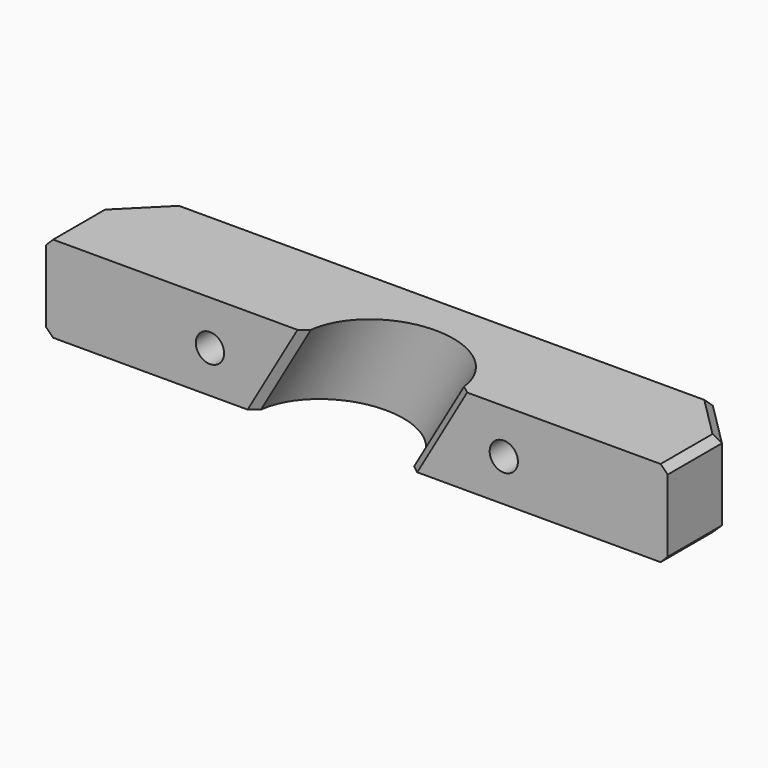
from build123d import *

# Parameters (mm, degrees)
F0_W         = 34.925
F0_H         = 12.7
F1_DEPTH     = 9.7155
F3_R         = 1.5875
F4_DEPTH     = 25.4
F5_SIZE      = 0.79375
F6_T1_DEPTH  = 34.2562991577
F7_SIZE      = 0.79375
F11_R        = 7.493
F12_DEPTH    = 50.8
F13_T1_DEPTH = 15.1455192093
F13_T3_DEPTH = 15.1455192093


# Not quite as in the source:
# - a fillet or chamfer that OpenCascade refuses, or shapes differently, is made with other operations: its cross-section is extruded or revolved along the edge and cut away or added


with BuildPart() as f1:
    # F0 (on Top) → F1 (new body)
    with BuildSketch(Plane.XY):
        with Locations((-17.4625, 6.35)):
            Rectangle(F0_W, F0_H)
        with Locations((17.4625, 6.35)):
            Rectangle(F0_W, F0_H)
    extrude(amount=F1_DEPTH)

    # F3 (on face) → F4 (cut)
    with BuildSketch(Plane(origin=(0, 12.7, 0), x_dir=(-1, 0, 0), z_dir=(0, 1, 0))):
        with Locations((16.51, 4.71678)):
            Circle(F3_R)
        with Locations((-16.51, 4.71678)):
            Circle(F3_R)
    extrude(amount=-F4_DEPTH, mode=Mode.SUBTRACT)

    # F5
    f5_edges = [f1.edges().sort_by_distance(p)[0] for p in [
        (-34.925, 6.35, 9.7155),
        (34.925, 6.35, 9.7155),
        (0, 12.7, 9.7155),
        (0, 12.7, 0),
        (-34.925, 6.35, 0),
        (34.925, 6.35, 0),
    ]]
    chamfer(f5_edges, length=F5_SIZE)

    # F6: chamfer of 5.08 on 2 edges, made by hand

    # F6_s2 → F6_t1 (cut)
    with BuildSketch(Plane.XY.offset(-12.2703995789)):
        Polygon((34.925, 7.62), (29.845, 12.7), (34.925, 12.7), align=None)
        Polygon((-34.925, 7.62), (-29.845, 12.7), (-34.925, 12.7), align=None)
    extrude(amount=F6_T1_DEPTH, mode=Mode.SUBTRACT)

    # F7
    f7_edges = [f1.edges().sort_by_distance(p)[0] for p in [
        (32.385, 10.16, 0),
        (32.385, 10.16, 9.7155),
        (-32.385, 10.16, 9.7155),
        (-32.385, 10.16, 0),
    ]]
    chamfer(f7_edges, length=F7_SIZE)

    # F11 (on face) → F12 (cut)
    with BuildSketch(Plane(origin=(-8.3875461679, 0, -14.5276561136), x_dir=(0.8660254038, 0, -0.5), z_dir=(0.5, 0, 0.8660254038))):
        with Locations((-2.3805295629, 0)):
            Circle(F11_R)
    extrude(amount=F12_DEPTH, mode=Mode.SUBTRACT)

    # F13: chamfer of 0.8001 on 2 edges, made by hand

    # F13_s2 → F13_t1 (cut)
    with BuildSketch(Plane(origin=(3.740760597, 0, 6.4791874129), x_dir=(0, 1, 0), z_dir=(-0.5, 0, -0.8660254038))):
        with BuildLine():
            Line((0, -10.6349433883), (0.7229081164, -9.8385757451))
            ThreePointArc((0.7229081164, -9.8385757451), (0.3732081581, -9.8642294948), (0, -9.8735295629))
            Line((0, -9.8735295629), (0, -10.6349433883))
        make_face()
    extrude(amount=F13_T1_DEPTH, mode=Mode.SUBTRACT)

    # F13_s4 → F13_t3 (cut)
    with BuildSketch(Plane(origin=(0.4940865594, 0, 0.8557830242), x_dir=(0, 1, 0), z_dir=(0.5, 0, 0.8660254038))):
        with BuildLine():
            Line((0, -5.8738842624), (0.7229081164, -5.0775166192))
            ThreePointArc((0.7229081164, -5.0775166192), (0.3732081581, -5.103170369), (0, -5.1124704371))
            Line((0, -5.1124704371), (0, -5.8738842624))
        make_face()
    extrude(amount=F13_T3_DEPTH, mode=Mode.SUBTRACT)


solid = f1.part
